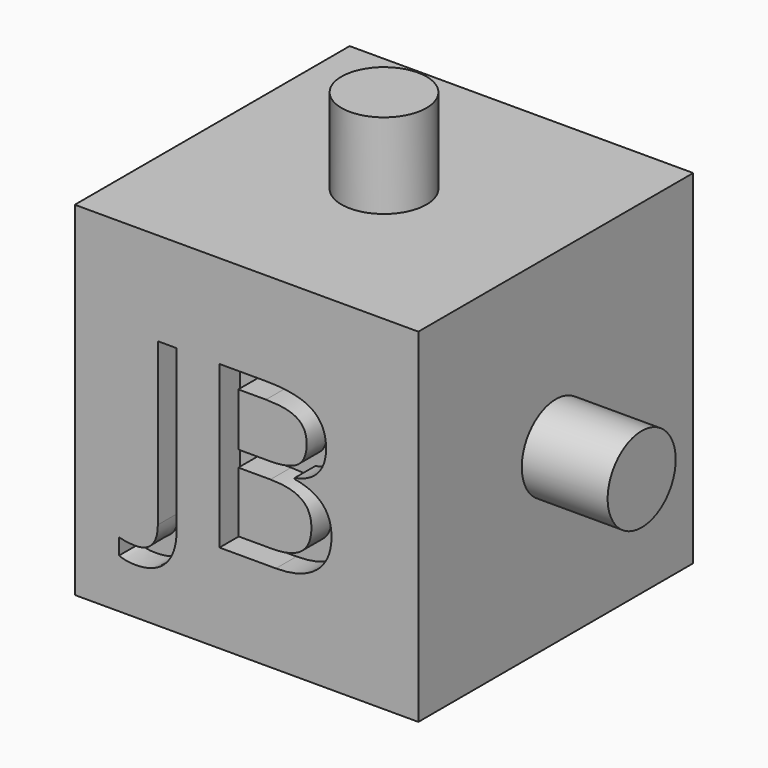
from build123d import *

# Parameters (mm, degrees)
F0_W         = 40
F0_H         = 40
F1_DEPTH     = 40
F2_TEXT_SIZE = 26.3601632064
F3_DEPTH     = 3
F4_R         = 4.95
F5_DEPTH     = 10
F6_R         = 4.95
F7_DEPTH     = 10
F8_R         = 4.95
F9_DEPTH     = 9.9
F10_R        = 4.95
F11_DEPTH    = 9.9


# Not quite as in the source:
# - Text() gives the source's letters only with a copy of the font that has no kerning and outlines rounded to 1/6400 em; it was checked with that copy


with BuildPart() as f1:
    # F0 (on Front) → F1 (new body)
    with BuildSketch(Plane.XZ):
        with Locations((20, 20)):
            Rectangle(F0_W, F0_H)
    extrude(amount=F1_DEPTH)

    # F2 (on face) → F3 (cut)
    with BuildSketch(Plane.XZ.offset(40)):
        with Locations((7.2234719992, 10.3394789621)):
            Text('JB', F2_TEXT_SIZE, font='Open Sans', text_align=(TextAlign.LEFT, TextAlign.BOTTOM))
    extrude(amount=-F3_DEPTH, mode=Mode.SUBTRACT)

    # F4 (on face) → F5 (join)
    with BuildSketch(Plane.YZ.offset(40)):
        with Locations((-20, 20)):
            Circle(F4_R)
    extrude(amount=F5_DEPTH)

    # F6 (on face) → F7 (join)
    with BuildSketch(Plane(origin=(0, 0, 0), x_dir=(0, -1, 0), z_dir=(-1, 0, 0))):
        with Locations((20, 20)):
            Circle(F6_R)
    extrude(amount=F7_DEPTH)

    # F8 (on face) → F9 (join)
    with BuildSketch(Plane(origin=(0, 0, 0), x_dir=(-1, 0, 0), z_dir=(0, 1, 0))):
        with Locations((-20, 20)):
            Circle(F8_R)
    extrude(amount=F9_DEPTH)

    # F10 (on face) → F11 (join)
    with BuildSketch(Plane.XY.offset(40)):
        with Locations((20, -20)):
            Circle(F10_R)
    extrude(amount=F11_DEPTH)


solid = f1.part
